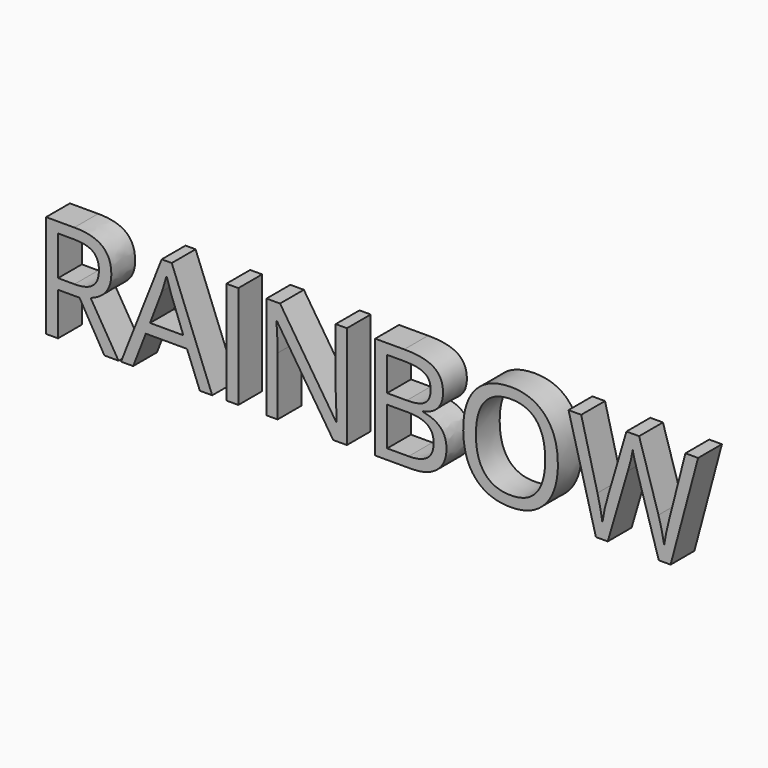
from build123d import *

# Parameters (mm, degrees)
F0_TEXT_SIZE = 122.9327379002
F1_DEPTH     = 25.4


# Not quite as in the source:
# - Text() gives the source's letters only with a copy of the font that has no kerning and outlines rounded to 1/6400 em; it was checked with that copy


with BuildPart() as f1:
    # F0 (on Front) → F1 (new body)
    with BuildSketch(Plane.XZ):
        with Locations((-132.4293762445, -48.5716946423)):
            Text('RAINBOW', F0_TEXT_SIZE, font='Open Sans', text_align=(TextAlign.LEFT, TextAlign.BOTTOM))
    extrude(amount=F1_DEPTH)


solid = f1.part
